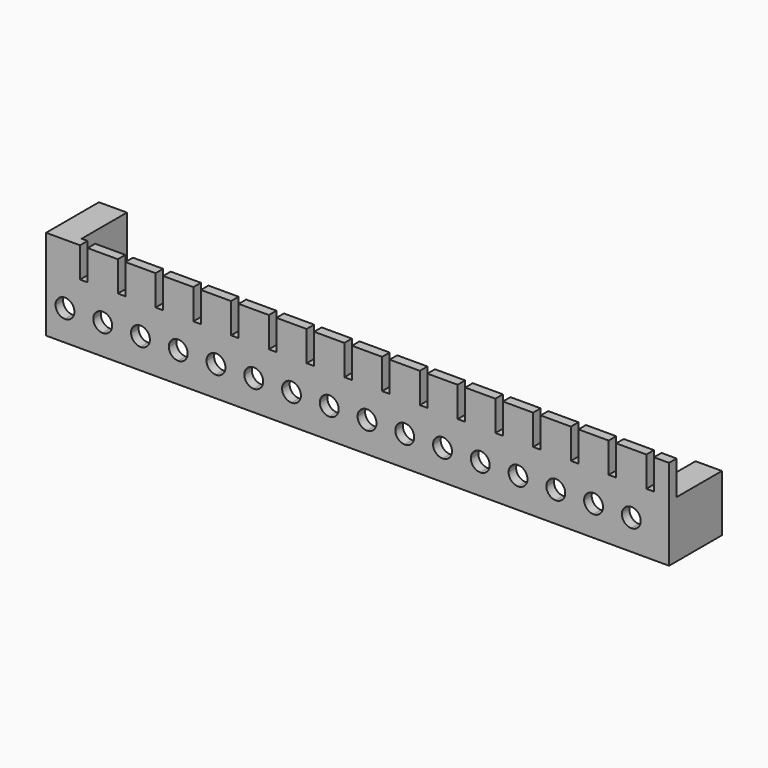
from build123d import *

# Parameters (mm, degrees)
F0_W     = 5.08
F0_H     = 10.16
F0_W_2   = 6.35
F1_DEPTH = 3.175
F2_W     = 8.8722240604
F2_H     = 19.05
F3_DEPTH = 19.05
F4_W     = 9.4110711813
F4_H     = 16.970772783
F5_DEPTH = 19.05


with BuildPart() as f1:
    # F0 (on Front) → F1 (new body)
    with BuildSketch(Plane.XZ):
        with Locations((-22.86, 10.16)):
            Rectangle(F0_W, F0_H)
        with Locations((-35.56, 10.16)):
            Rectangle(F0_W, F0_H)
        with BuildLine():
            Line((31.75, -5.08), (31.75, -15.24))
            Line((31.75, -15.24), (38.1, -15.24))
            Line((38.1, -15.24), (38.1, -8.255))
            ThreePointArc((38.1, -8.255), (35.8549359697, -7.3250640303), (34.925, -5.08))
            Line((34.925, -5.08), (31.75, -5.08))
        make_face()
        with BuildLine():
            Line((53.975, -5.08), (57.15, -5.08))
            Line((57.15, -5.08), (57.15, 5.08))
            Line((57.15, 5.08), (55.88, 5.08))
            Line((55.88, 5.08), (50.8, 5.08))
            Line((50.8, 5.08), (50.8, -1.905))
            ThreePointArc((50.8, -1.905), (53.0450640303, -2.8349359697), (53.975, -5.08))
        make_face()
        with Locations((66.04, 10.16)):
            Rectangle(F0_W, F0_H)
        with BuildLine():
            Line((-83.82, 5.08), (-88.9, 5.08))
            Line((-88.9, 5.08), (-88.9, -1.905))
            ThreePointArc((-88.9, -1.905), (-86.6549359697, -2.8349359697), (-85.725, -5.08))
            Line((-85.725, -5.08), (-82.55, -5.08))
            Line((-82.55, -5.08), (-82.55, 5.08))
            Line((-82.55, 5.08), (-83.82, 5.08))
        make_face()
        with BuildLine():
            Line((-57.15, 5.08), (-57.15, -5.08))
            Line((-57.15, -5.08), (-53.975, -5.08))
            ThreePointArc((-53.975, -5.08), (-53.0450640303, -2.8349359697), (-50.8, -1.905))
            Line((-50.8, -1.905), (-50.8, 5.08))
            Line((-50.8, 5.08), (-55.88, 5.08))
            Line((-55.88, 5.08), (-57.15, 5.08))
        make_face()
        with BuildLine():
            Line((-44.45, -5.08), (-44.45, -15.24))
            Line((-44.45, -15.24), (-38.1, -15.24))
            Line((-38.1, -15.24), (-38.1, -8.255))
            ThreePointArc((-38.1, -8.255), (-40.3450640303, -7.3250640303), (-41.275, -5.08))
            Line((-41.275, -5.08), (-44.45, -5.08))
        make_face()
        with BuildLine():
            Line((-47.625, -5.08), (-44.45, -5.08))
            Line((-44.45, -5.08), (-44.45, 5.08))
            Line((-44.45, 5.08), (-45.72, 5.08))
            Line((-45.72, 5.08), (-50.8, 5.08))
            Line((-50.8, 5.08), (-50.8, -1.905))
            ThreePointArc((-50.8, -1.905), (-48.5549359697, -2.8349359697), (-47.625, -5.08))
        make_face()
        with BuildLine():
            Line((-63.5, -8.255), (-63.5, -15.24))
            Line((-63.5, -15.24), (-57.15, -15.24))
            Line((-57.15, -15.24), (-57.15, -5.08))
            Line((-57.15, -5.08), (-60.325, -5.08))
            ThreePointArc((-60.325, -5.08), (-61.2549359697, -7.3250640303), (-63.5, -8.255))
        make_face()
        with BuildLine():
            Line((-76.2, -8.255), (-76.2, -15.24))
            Line((-76.2, -15.24), (-69.85, -15.24))
            Line((-69.85, -15.24), (-69.85, -5.08))
            Line((-69.85, -5.08), (-73.025, -5.08))
            ThreePointArc((-73.025, -5.08), (-73.9549359697, -7.3250640303), (-76.2, -8.255))
        make_face()
        with BuildLine():
            Line((3.175, -5.08), (6.35, -5.08))
            Line((6.35, -5.08), (6.35, 5.08))
            Line((6.35, 5.08), (5.08, 5.08))
            Line((5.08, 5.08), (0, 5.08))
            Line((0, 5.08), (0, -1.905))
            ThreePointArc((0, -1.905), (2.2450640303, -2.8349359697), (3.175, -5.08))
        make_face()
        with Locations((78.74, 10.16)):
            Rectangle(F0_W, F0_H)
        with BuildLine():
            Line((-69.85, -5.08), (-69.85, -15.24))
            Line((-69.85, -15.24), (-63.5, -15.24))
            Line((-63.5, -15.24), (-63.5, -8.255))
            ThreePointArc((-63.5, -8.255), (-65.7450640303, -7.3250640303), (-66.675, -5.08))
            Line((-66.675, -5.08), (-69.85, -5.08))
        make_face()
        with Locations((2.54, 10.16)):
            Rectangle(F0_W, F0_H)
        with BuildLine():
            Line((38.1, -8.255), (38.1, -15.24))
            Line((38.1, -15.24), (44.45, -15.24))
            Line((44.45, -15.24), (44.45, -5.08))
            Line((44.45, -5.08), (41.275, -5.08))
            ThreePointArc((41.275, -5.08), (40.3450640303, -7.3250640303), (38.1, -8.255))
        make_face()
        with Locations((10.16, 10.16)):
            Rectangle(F0_W, F0_H)
        with Locations((22.86, 10.16)):
            Rectangle(F0_W, F0_H)
        with BuildLine():
            Line((12.7, -8.255), (12.7, -15.24))
            Line((12.7, -15.24), (19.05, -15.24))
            Line((19.05, -15.24), (19.05, -5.08))
            Line((19.05, -5.08), (15.875, -5.08))
            ThreePointArc((15.875, -5.08), (14.9450640303, -7.3250640303), (12.7, -8.255))
        make_face()
        with BuildLine():
            Line((25.4, -8.255), (25.4, -15.24))
            Line((25.4, -15.24), (31.75, -15.24))
            Line((31.75, -15.24), (31.75, -5.08))
            Line((31.75, -5.08), (28.575, -5.08))
            ThreePointArc((28.575, -5.08), (27.6450640303, -7.3250640303), (25.4, -8.255))
        make_face()
        with BuildLine():
            Line((15.875, -5.08), (19.05, -5.08))
            Line((19.05, -5.08), (19.05, 5.08))
            Line((19.05, 5.08), (17.78, 5.08))
            Line((17.78, 5.08), (12.7, 5.08))
            Line((12.7, 5.08), (12.7, -1.905))
            ThreePointArc((12.7, -1.905), (14.9450640303, -2.8349359697), (15.875, -5.08))
        make_face()
        with BuildLine():
            Line((-58.42, 5.08), (-63.5, 5.08))
            Line((-63.5, 5.08), (-63.5, -1.905))
            ThreePointArc((-63.5, -1.905), (-61.2549359697, -2.8349359697), (-60.325, -5.08))
            Line((-60.325, -5.08), (-57.15, -5.08))
            Line((-57.15, -5.08), (-57.15, 5.08))
            Line((-57.15, 5.08), (-58.42, 5.08))
        make_face()
        with BuildLine():
            Line((-71.12, 5.08), (-76.2, 5.08))
            Line((-76.2, 5.08), (-76.2, -1.905))
            ThreePointArc((-76.2, -1.905), (-73.9549359697, -2.8349359697), (-73.025, -5.08))
            Line((-73.025, -5.08), (-69.85, -5.08))
            Line((-69.85, -5.08), (-69.85, 5.08))
            Line((-69.85, 5.08), (-71.12, 5.08))
        make_face()
        with Locations((-2.54, 10.16)):
            Rectangle(F0_W, F0_H)
        with Locations((91.44, 10.16)):
            Rectangle(F0_W, F0_H)
        with BuildLine():
            Line((28.575, -5.08), (31.75, -5.08))
            Line((31.75, -5.08), (31.75, 5.08))
            Line((31.75, 5.08), (30.48, 5.08))
            Line((30.48, 5.08), (25.4, 5.08))
            Line((25.4, 5.08), (25.4, -1.905))
            ThreePointArc((25.4, -1.905), (27.6450640303, -2.8349359697), (28.575, -5.08))
        make_face()
        with BuildLine():
            Line((57.15, -5.08), (57.15, -15.24))
            Line((57.15, -15.24), (63.5, -15.24))
            Line((63.5, -15.24), (63.5, -8.255))
            ThreePointArc((63.5, -8.255), (61.2549359697, -7.3250640303), (60.325, -5.08))
            Line((60.325, -5.08), (57.15, -5.08))
        make_face()
        with Locations((-78.74, 10.16)):
            Rectangle(F0_W, F0_H)
        with BuildLine():
            Line((50.8, -8.255), (50.8, -15.24))
            Line((50.8, -15.24), (57.15, -15.24))
            Line((57.15, -15.24), (57.15, -5.08))
            Line((57.15, -5.08), (53.975, -5.08))
            ThreePointArc((53.975, -5.08), (53.0450640303, -7.3250640303), (50.8, -8.255))
        make_face()
        with BuildLine():
            Line((-44.45, 5.08), (-44.45, -5.08))
            Line((-44.45, -5.08), (-41.275, -5.08))
            ThreePointArc((-41.275, -5.08), (-40.3450640303, -2.8349359697), (-38.1, -1.905))
            Line((-38.1, -1.905), (-38.1, 5.08))
            Line((-38.1, 5.08), (-43.18, 5.08))
            Line((-43.18, 5.08), (-44.45, 5.08))
        make_face()
        with BuildLine():
            Line((57.15, 5.08), (57.15, -5.08))
            Line((57.15, -5.08), (60.325, -5.08))
            ThreePointArc((60.325, -5.08), (61.2549359697, -2.8349359697), (63.5, -1.905))
            Line((63.5, -1.905), (63.5, 5.08))
            Line((63.5, 5.08), (58.42, 5.08))
            Line((58.42, 5.08), (57.15, 5.08))
        make_face()
        with BuildLine():
            Line((-92.075, -5.08), (-95.25, -5.08))
            Line((-95.25, -5.08), (-95.25, -15.24))
            Line((-95.25, -15.24), (-88.9, -15.24))
            Line((-88.9, -15.24), (-88.9, -8.255))
            ThreePointArc((-88.9, -8.255), (-91.1450640303, -7.3250640303), (-92.075, -5.08))
        make_face()
        with BuildLine():
            Line((41.275, -5.08), (44.45, -5.08))
            Line((44.45, -5.08), (44.45, 5.08))
            Line((44.45, 5.08), (43.18, 5.08))
            Line((43.18, 5.08), (38.1, 5.08))
            Line((38.1, 5.08), (38.1, -1.905))
            ThreePointArc((38.1, -1.905), (40.3450640303, -2.8349359697), (41.275, -5.08))
        make_face()
        with BuildLine():
            Line((44.45, 5.08), (44.45, -5.08))
            Line((44.45, -5.08), (47.625, -5.08))
            ThreePointArc((47.625, -5.08), (48.5549359697, -2.8349359697), (50.8, -1.905))
            Line((50.8, -1.905), (50.8, 5.08))
            Line((50.8, 5.08), (45.72, 5.08))
            Line((45.72, 5.08), (44.45, 5.08))
        make_face()
        with Locations((-86.36, 10.16)):
            Rectangle(F0_W, F0_H)
        with BuildLine():
            Line((101.6, -8.255), (101.6, -15.24))
            Line((101.6, -15.24), (107.95, -15.24))
            Line((107.95, -15.24), (107.95, 5.08))
            Line((107.95, 5.08), (106.68, 5.08))
            Line((106.68, 5.08), (106.68, 15.24))
            Line((106.68, 15.24), (101.6, 15.24))
            Line((101.6, 15.24), (101.6, -1.905))
            ThreePointArc((101.6, -1.905), (103.8450640303, -2.8349359697), (104.775, -5.08))
            ThreePointArc((104.775, -5.08), (103.8450640303, -7.3250640303), (101.6, -8.255))
        make_face()
        with BuildLine():
            Line((-82.55, -5.08), (-85.725, -5.08))
            ThreePointArc((-85.725, -5.08), (-86.6549359697, -7.3250640303), (-88.9, -8.255))
            Line((-88.9, -8.255), (-88.9, -15.24))
            Line((-88.9, -15.24), (-82.55, -15.24))
            Line((-82.55, -15.24), (-82.55, -5.08))
        make_face()
        with BuildLine():
            Line((-57.15, -5.08), (-57.15, -15.24))
            Line((-57.15, -15.24), (-50.8, -15.24))
            Line((-50.8, -15.24), (-50.8, -8.255))
            ThreePointArc((-50.8, -8.255), (-53.0450640303, -7.3250640303), (-53.975, -5.08))
            Line((-53.975, -5.08), (-57.15, -5.08))
        make_face()
        with BuildLine():
            Line((31.75, 5.08), (31.75, -5.08))
            Line((31.75, -5.08), (34.925, -5.08))
            ThreePointArc((34.925, -5.08), (35.8549359697, -2.8349359697), (38.1, -1.905))
            Line((38.1, -1.905), (38.1, 5.08))
            Line((38.1, 5.08), (33.02, 5.08))
            Line((33.02, 5.08), (31.75, 5.08))
        make_face()
        with BuildLine():
            Line((44.45, -5.08), (44.45, -15.24))
            Line((44.45, -15.24), (50.8, -15.24))
            Line((50.8, -15.24), (50.8, -8.255))
            ThreePointArc((50.8, -8.255), (48.5549359697, -7.3250640303), (47.625, -5.08))
            Line((47.625, -5.08), (44.45, -5.08))
        make_face()
        with BuildLine():
            Line((-68.58, 5.08), (-69.85, 5.08))
            Line((-69.85, 5.08), (-69.85, -5.08))
            Line((-69.85, -5.08), (-66.675, -5.08))
            ThreePointArc((-66.675, -5.08), (-65.7450640303, -2.8349359697), (-63.5, -1.905))
            Line((-63.5, -1.905), (-63.5, 5.08))
            Line((-63.5, 5.08), (-68.58, 5.08))
        make_face()
        with Locations((15.24, 10.16)):
            Rectangle(F0_W, F0_H)
        with Locations((-10.16, 10.16)):
            Rectangle(F0_W, F0_H)
        with BuildLine():
            Line((-6.35, -5.08), (-6.35, -15.24))
            Line((-6.35, -15.24), (0, -15.24))
            Line((0, -15.24), (0, -8.255))
            ThreePointArc((0, -8.255), (-2.2450640303, -7.3250640303), (-3.175, -5.08))
            Line((-3.175, -5.08), (-6.35, -5.08))
        make_face()
        with BuildLine():
            Line((-50.8, -8.255), (-50.8, -15.24))
            Line((-50.8, -15.24), (-44.45, -15.24))
            Line((-44.45, -15.24), (-44.45, -5.08))
            Line((-44.45, -5.08), (-47.625, -5.08))
            ThreePointArc((-47.625, -5.08), (-48.5549359697, -7.3250640303), (-50.8, -8.255))
        make_face()
        with BuildLine():
            Line((-88.9, 5.08), (-95.25, 5.08))
            Line((-95.25, 5.08), (-95.25, -5.08))
            Line((-95.25, -5.08), (-92.075, -5.08))
            ThreePointArc((-92.075, -5.08), (-91.1450640303, -2.8349359697), (-88.9, -1.905))
            Line((-88.9, -1.905), (-88.9, 5.08))
        make_face()
        with BuildLine():
            Line((0, -8.255), (0, -15.24))
            Line((0, -15.24), (6.35, -15.24))
            Line((6.35, -15.24), (6.35, -5.08))
            Line((6.35, -5.08), (3.175, -5.08))
            ThreePointArc((3.175, -5.08), (2.2450640303, -7.3250640303), (0, -8.255))
        make_face()
        Polygon((107.95, 5.08), (107.95, -15.24), (114.3, -15.24), (114.3, 15.24), (109.22, 15.24), (109.22, 5.08), align=None)
        with BuildLine():
            Line((-34.925, -5.08), (-31.75, -5.08))
            Line((-31.75, -5.08), (-31.75, 5.08))
            Line((-31.75, 5.08), (-33.02, 5.08))
            Line((-33.02, 5.08), (-38.1, 5.08))
            Line((-38.1, 5.08), (-38.1, -1.905))
            ThreePointArc((-38.1, -1.905), (-35.8549359697, -2.8349359697), (-34.925, -5.08))
        make_face()
        with BuildLine():
            Line((63.5, -8.255), (63.5, -15.24))
            Line((63.5, -15.24), (69.85, -15.24))
            Line((69.85, -15.24), (69.85, -5.08))
            Line((69.85, -5.08), (66.675, -5.08))
            ThreePointArc((66.675, -5.08), (65.7450640303, -7.3250640303), (63.5, -8.255))
        make_face()
        with BuildLine():
            Line((-38.1, -8.255), (-38.1, -15.24))
            Line((-38.1, -15.24), (-31.75, -15.24))
            Line((-31.75, -15.24), (-31.75, -5.08))
            Line((-31.75, -5.08), (-34.925, -5.08))
            ThreePointArc((-34.925, -5.08), (-35.8549359697, -7.3250640303), (-38.1, -8.255))
        make_face()
        with Locations((-40.64, 10.16)):
            Rectangle(F0_W, F0_H)
        with Locations((60.96, 10.16)):
            Rectangle(F0_W, F0_H)
        with BuildLine():
            Line((6.35, -5.08), (6.35, -15.24))
            Line((6.35, -15.24), (12.7, -15.24))
            Line((12.7, -15.24), (12.7, -8.255))
            ThreePointArc((12.7, -8.255), (10.4549359697, -7.3250640303), (9.525, -5.08))
            Line((9.525, -5.08), (6.35, -5.08))
        make_face()
        with BuildLine():
            Line((95.25, -5.08), (95.25, -15.24))
            Line((95.25, -15.24), (101.6, -15.24))
            Line((101.6, -15.24), (101.6, -8.255))
            ThreePointArc((101.6, -8.255), (98.425, -5.08), (101.6, -1.905))
            Line((101.6, -1.905), (101.6, 15.24))
            Line((101.6, 15.24), (96.52, 15.24))
            Line((96.52, 15.24), (96.52, 5.08))
            Line((96.52, 5.08), (95.25, 5.08))
            Line((95.25, 5.08), (95.25, -5.08))
        make_face()
        with BuildLine():
            Line((6.35, 5.08), (6.35, -5.08))
            Line((6.35, -5.08), (9.525, -5.08))
            ThreePointArc((9.525, -5.08), (10.4549359697, -2.8349359697), (12.7, -1.905))
            Line((12.7, -1.905), (12.7, 5.08))
            Line((12.7, 5.08), (7.62, 5.08))
            Line((7.62, 5.08), (6.35, 5.08))
        make_face()
        with BuildLine():
            Line((66.675, -5.08), (69.85, -5.08))
            Line((69.85, -5.08), (69.85, 5.08))
            Line((69.85, 5.08), (68.58, 5.08))
            Line((68.58, 5.08), (63.5, 5.08))
            Line((63.5, 5.08), (63.5, -1.905))
            ThreePointArc((63.5, -1.905), (65.7450640303, -2.8349359697), (66.675, -5.08))
        make_face()
        with Locations((27.94, 10.16)):
            Rectangle(F0_W, F0_H)
        with Locations((-73.66, 10.16)):
            Rectangle(F0_W, F0_H)
        with Locations((-92.075, 10.16)):
            Rectangle(F0_W_2, F0_H)
        with BuildLine():
            Line((-31.75, 5.08), (-31.75, -5.08))
            Line((-31.75, -5.08), (-28.575, -5.08))
            ThreePointArc((-28.575, -5.08), (-27.6450640303, -2.8349359697), (-25.4, -1.905))
            Line((-25.4, -1.905), (-25.4, 5.08))
            Line((-25.4, 5.08), (-30.48, 5.08))
            Line((-30.48, 5.08), (-31.75, 5.08))
        make_face()
        with BuildLine():
            Line((69.85, -5.08), (69.85, -15.24))
            Line((69.85, -15.24), (76.2, -15.24))
            Line((76.2, -15.24), (76.2, -8.255))
            ThreePointArc((76.2, -8.255), (73.9549359697, -7.3250640303), (73.025, -5.08))
            Line((73.025, -5.08), (69.85, -5.08))
        make_face()
        with Locations((-27.94, 10.16)):
            Rectangle(F0_W, F0_H)
        with Locations((73.66, 10.16)):
            Rectangle(F0_W, F0_H)
        with BuildLine():
            Line((92.075, -5.08), (95.25, -5.08))
            Line((95.25, -5.08), (95.25, 5.08))
            Line((95.25, 5.08), (93.98, 5.08))
            Line((93.98, 5.08), (88.9, 5.08))
            Line((88.9, 5.08), (88.9, -1.905))
            ThreePointArc((88.9, -1.905), (91.1450640303, -2.8349359697), (92.075, -5.08))
        make_face()
        with BuildLine():
            Line((-31.75, -5.08), (-31.75, -15.24))
            Line((-31.75, -15.24), (-25.4, -15.24))
            Line((-25.4, -15.24), (-25.4, -8.255))
            ThreePointArc((-25.4, -8.255), (-27.6450640303, -7.3250640303), (-28.575, -5.08))
            Line((-28.575, -5.08), (-31.75, -5.08))
        make_face()
        with BuildLine():
            Line((69.85, 5.08), (69.85, -5.08))
            Line((69.85, -5.08), (73.025, -5.08))
            ThreePointArc((73.025, -5.08), (73.9549359697, -2.8349359697), (76.2, -1.905))
            Line((76.2, -1.905), (76.2, 5.08))
            Line((76.2, 5.08), (71.12, 5.08))
            Line((71.12, 5.08), (69.85, 5.08))
        make_face()
        with Locations((35.56, 10.16)):
            Rectangle(F0_W, F0_H)
        with Locations((-66.04, 10.16)):
            Rectangle(F0_W, F0_H)
        with BuildLine():
            Line((79.375, -5.08), (82.55, -5.08))
            Line((82.55, -5.08), (82.55, 5.08))
            Line((82.55, 5.08), (81.28, 5.08))
            Line((81.28, 5.08), (76.2, 5.08))
            Line((76.2, 5.08), (76.2, -1.905))
            ThreePointArc((76.2, -1.905), (78.4450640303, -2.8349359697), (79.375, -5.08))
        make_face()
        with BuildLine():
            Line((-12.7, -8.255), (-12.7, -15.24))
            Line((-12.7, -15.24), (-6.35, -15.24))
            Line((-6.35, -15.24), (-6.35, -5.08))
            Line((-6.35, -5.08), (-9.525, -5.08))
            ThreePointArc((-9.525, -5.08), (-10.4549359697, -7.3250640303), (-12.7, -8.255))
        make_face()
        with BuildLine():
            Line((88.9, -8.255), (88.9, -15.24))
            Line((88.9, -15.24), (95.25, -15.24))
            Line((95.25, -15.24), (95.25, -5.08))
            Line((95.25, -5.08), (92.075, -5.08))
            ThreePointArc((92.075, -5.08), (91.1450640303, -7.3250640303), (88.9, -8.255))
        make_face()
        with BuildLine():
            Line((-9.525, -5.08), (-6.35, -5.08))
            Line((-6.35, -5.08), (-6.35, 5.08))
            Line((-6.35, 5.08), (-7.62, 5.08))
            Line((-7.62, 5.08), (-12.7, 5.08))
            Line((-12.7, 5.08), (-12.7, -1.905))
            ThreePointArc((-12.7, -1.905), (-10.4549359697, -2.8349359697), (-9.525, -5.08))
        make_face()
        with Locations((-48.26, 10.16)):
            Rectangle(F0_W, F0_H)
        with Locations((53.34, 10.16)):
            Rectangle(F0_W, F0_H)
        with Locations((40.64, 10.16)):
            Rectangle(F0_W, F0_H)
        with Locations((-60.96, 10.16)):
            Rectangle(F0_W, F0_H)
        with BuildLine():
            Line((-22.225, -5.08), (-19.05, -5.08))
            Line((-19.05, -5.08), (-19.05, 5.08))
            Line((-19.05, 5.08), (-20.32, 5.08))
            Line((-20.32, 5.08), (-25.4, 5.08))
            Line((-25.4, 5.08), (-25.4, -1.905))
            ThreePointArc((-25.4, -1.905), (-23.1549359697, -2.8349359697), (-22.225, -5.08))
        make_face()
        with BuildLine():
            Line((76.2, -8.255), (76.2, -15.24))
            Line((76.2, -15.24), (82.55, -15.24))
            Line((82.55, -15.24), (82.55, -5.08))
            Line((82.55, -5.08), (79.375, -5.08))
            ThreePointArc((79.375, -5.08), (78.4450640303, -7.3250640303), (76.2, -8.255))
        make_face()
        with BuildLine():
            Line((-25.4, -8.255), (-25.4, -15.24))
            Line((-25.4, -15.24), (-19.05, -15.24))
            Line((-19.05, -15.24), (-19.05, -5.08))
            Line((-19.05, -5.08), (-22.225, -5.08))
            ThreePointArc((-22.225, -5.08), (-23.1549359697, -7.3250640303), (-25.4, -8.255))
        make_face()
        with Locations((-15.24, 10.16)):
            Rectangle(F0_W, F0_H)
        with Locations((48.26, 10.16)):
            Rectangle(F0_W, F0_H)
        with Locations((-53.34, 10.16)):
            Rectangle(F0_W, F0_H)
        with Locations((86.36, 10.16)):
            Rectangle(F0_W, F0_H)
        with BuildLine():
            Line((19.05, -5.08), (19.05, -15.24))
            Line((19.05, -15.24), (25.4, -15.24))
            Line((25.4, -15.24), (25.4, -8.255))
            ThreePointArc((25.4, -8.255), (23.1549359697, -7.3250640303), (22.225, -5.08))
            Line((22.225, -5.08), (19.05, -5.08))
        make_face()
        with BuildLine():
            Line((-19.05, 5.08), (-19.05, -5.08))
            Line((-19.05, -5.08), (-15.875, -5.08))
            ThreePointArc((-15.875, -5.08), (-14.9450640303, -2.8349359697), (-12.7, -1.905))
            Line((-12.7, -1.905), (-12.7, 5.08))
            Line((-12.7, 5.08), (-17.78, 5.08))
            Line((-17.78, 5.08), (-19.05, 5.08))
        make_face()
        with BuildLine():
            Line((-79.375, -5.08), (-82.55, -5.08))
            Line((-82.55, -5.08), (-82.55, -15.24))
            Line((-82.55, -15.24), (-76.2, -15.24))
            Line((-76.2, -15.24), (-76.2, -8.255))
            ThreePointArc((-76.2, -8.255), (-78.4450640303, -7.3250640303), (-79.375, -5.08))
        make_face()
        with BuildLine():
            Line((82.55, -5.08), (82.55, -15.24))
            Line((82.55, -15.24), (88.9, -15.24))
            Line((88.9, -15.24), (88.9, -8.255))
            ThreePointArc((88.9, -8.255), (86.6549359697, -7.3250640303), (85.725, -5.08))
            Line((85.725, -5.08), (82.55, -5.08))
        make_face()
        with BuildLine():
            Line((-19.05, -5.08), (-19.05, -15.24))
            Line((-19.05, -15.24), (-12.7, -15.24))
            Line((-12.7, -15.24), (-12.7, -8.255))
            ThreePointArc((-12.7, -8.255), (-14.9450640303, -7.3250640303), (-15.875, -5.08))
            Line((-15.875, -5.08), (-19.05, -5.08))
        make_face()
        with BuildLine():
            Line((19.05, 5.08), (19.05, -5.08))
            Line((19.05, -5.08), (22.225, -5.08))
            ThreePointArc((22.225, -5.08), (23.1549359697, -2.8349359697), (25.4, -1.905))
            Line((25.4, -1.905), (25.4, 5.08))
            Line((25.4, 5.08), (20.32, 5.08))
            Line((20.32, 5.08), (19.05, 5.08))
        make_face()
        with BuildLine():
            Line((-81.28, 5.08), (-82.55, 5.08))
            Line((-82.55, 5.08), (-82.55, -5.08))
            Line((-82.55, -5.08), (-79.375, -5.08))
            ThreePointArc((-79.375, -5.08), (-78.4450640303, -2.8349359697), (-76.2, -1.905))
            Line((-76.2, -1.905), (-76.2, 5.08))
            Line((-76.2, 5.08), (-81.28, 5.08))
        make_face()
        with BuildLine():
            Line((82.55, 5.08), (82.55, -5.08))
            Line((82.55, -5.08), (85.725, -5.08))
            ThreePointArc((85.725, -5.08), (86.6549359697, -2.8349359697), (88.9, -1.905))
            Line((88.9, -1.905), (88.9, 5.08))
            Line((88.9, 5.08), (83.82, 5.08))
            Line((83.82, 5.08), (82.55, 5.08))
        make_face()
        with BuildLine():
            Line((-6.35, 5.08), (-6.35, -5.08))
            Line((-6.35, -5.08), (-3.175, -5.08))
            ThreePointArc((-3.175, -5.08), (-2.2450640303, -2.8349359697), (0, -1.905))
            Line((0, -1.905), (0, 5.08))
            Line((0, 5.08), (-5.08, 5.08))
            Line((-5.08, 5.08), (-6.35, 5.08))
        make_face()
    extrude(amount=F1_DEPTH)

    # F2 (on face) → F3 (join)
    with BuildSketch(Plane(origin=(0, 0, 0), x_dir=(-1, 0, 0), z_dir=(0, 1, 0))):
        with Locations((-109.8638879698, -5.715)):
            Rectangle(F2_W, F2_H)
    extrude(amount=F3_DEPTH)

    # F4 (on face) → F5 (join)
    with BuildSketch(Plane(origin=(0, 0, 0), x_dir=(-1, 0, 0), z_dir=(0, 1, 0))):
        with Locations((90.5444644094, 6.7546136085)):
            Rectangle(F4_W, F4_H)
    extrude(amount=F5_DEPTH)


solid = f1.part
